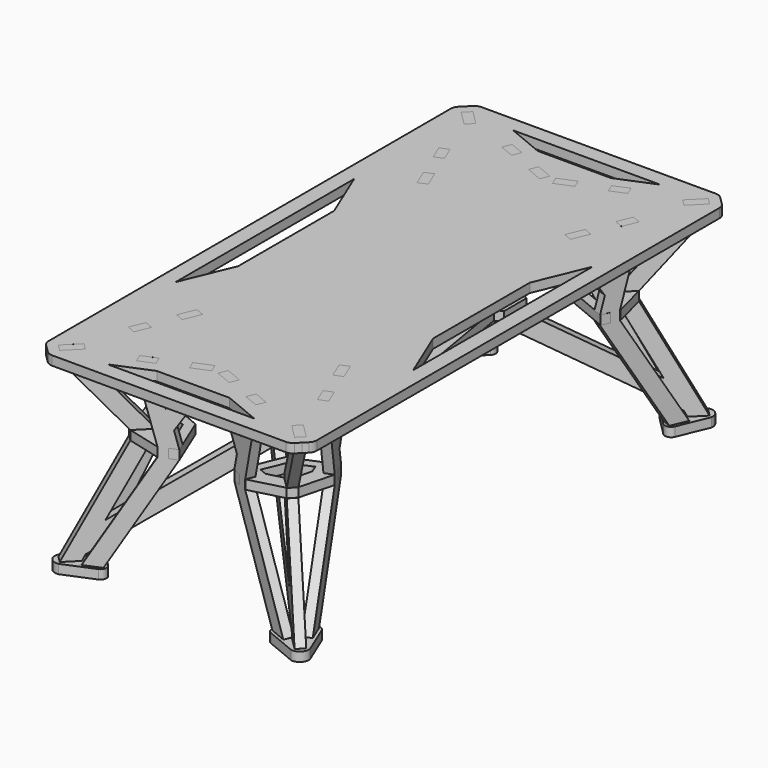
from build123d import *

# Parameters (mm, degrees)
F3_DEPTH  = 9.525
F6_DEPTH  = 9.525
F9_DEPTH  = 9.525
F12_DEPTH = 19.05
F15_DEPTH = 9.525
F18_DEPTH = 9.525
F21_DEPTH = 9.525
F24_DEPTH = 19.05
F25_DEPTH = 19.05
F26_DEPTH = 19.05
F27_DEPTH = 19.05
F28_DEPTH = 19.05
F31_DEPTH = 9.525
F34_DEPTH = 9.525
F37_DEPTH = 9.525
F40_DEPTH = 9.525
F43_DEPTH = 9.525
F46_DEPTH = 9.525
F49_DEPTH = 19.05
F52_DEPTH = 19.05
F55_DEPTH = 19.05
F58_DEPTH = 19.05


# Not quite as in the source:
# - a feature names something its author has since deleted; it is built from what else it names


with BuildPart() as f3:
    # F2 (on face) → F3 (new body, symmetric)
    with BuildSketch(Plane(origin=(0.1198709265, -0.1198709265, 0), x_dir=(0.7071067812, 0.7071067812, 0), z_dir=(0.7071067812, -0.7071067812, 0))):
        Polygon((72.1438338904, -0.0049185293), (72.1438338904, 19.0450814707), (76.4979425715, 19.0450814707), (82.66578851, 30.7838885104), (431.821256876, 234.9450814707), (431.821256876, 253.9950814707), (404.6548892498, 253.9950814707), (404.6548892498, 234.9450814707), (385.6048892498, 234.9450814707), (385.6048892498, 253.9950814707), (360.1152509125, 253.9950814707), (360.1152509125, 234.9450814707), (115.2544208988, 91.7679478036), (191.7653489945, 234.9450814707), (191.7653489945, 260.9125323174), (101.4276913023, 365.3266918993), (101.4276913023, 387.3450814707), (82.3776913023, 387.3450814707), (82.3776913023, 406.3950814707), (40.3938338904, 406.3950814707), (40.3938338904, 387.3450814707), (155.766372457, 253.9950814707), (173.7658607257, 253.9950814707), (173.7658607257, 234.9450814707), (155.766372457, 234.9450814707), (40.3938338904, 19.0450814707), (40.3938338904, -0.0049185293), align=None)
    extrude(amount=F3_DEPTH, both=True)


with BuildPart() as f6:
    # F5 (on line) → F6 (new body, symmetric)
    with BuildSketch(Plane(origin=(-6.0751025032, 14.6665948559, 0), x_dir=(-0.9238795325, -0.3826834324, 0), z_dir=(-0.3826834324, 0.9238795325, 0))):
        Polygon((-114.9103235555, 19.0475704348), (-109.7184195119, 19.0475704348), (-109.7184195119, -0.0024295652), (-77.970899542, -0.0024295652), (-77.970899542, 19.0475704348), (-206.3556462526, 234.9475704348), (-206.3556462526, 253.9975704348), (-170.8678305149, 387.3475704348), (-170.8678305149, 406.3975704348), (-203.7229094406, 406.3975704348), (-203.7229094406, 387.3475704348), (-210.0729094406, 387.3475704348), (-210.0729094406, 363.4866344375), (-220.3803230208, 324.7552114874), (-254.0578127939, 377.4178575907), (-254.0578127939, 387.3475704348), (-260.4078127939, 387.3475704348), (-260.4078127939, 406.3975704348), (-298.0948572889, 406.3975704348), (-298.0948572889, 387.3475704348), (-234.3391501722, 287.6505840032), (-243.2950702662, 253.9975704348), (-224.8253582594, 253.9975704348), (-224.8253582594, 234.9475704348), (-243.2950702662, 234.9475704348), align=None)
    extrude(amount=F6_DEPTH, both=True)


with BuildPart() as f9:
    # F8 (on line) → F9 (new body, symmetric)
    with BuildSketch(Plane(origin=(14.6666075026, -6.0751077416, 0), x_dir=(0.3826834324, 0.9238795325, 0), z_dir=(0.9238795325, -0.3826834324, 0))):
        Polygon((206.0561226085, 253.999334064), (206.0561226085, 234.949334064), (77.6713758978, 19.049334064), (77.6713758978, -0.000665936), (109.4188958678, -0.000665936), (109.4188958678, 19.049334064), (114.6107999114, 19.049334064), (242.995546622, 234.949334064), (224.5258346153, 234.949334064), (224.5258346153, 253.999334064), (242.995546622, 253.999334064), (234.039626528, 287.6523476325), (297.7953336448, 387.349334064), (297.7953336448, 406.399334064), (260.1082891497, 406.399334064), (260.1082891497, 387.349334064), (253.7582891497, 387.349334064), (253.7582891497, 377.41962122), (220.0807993766, 324.7569751166), (209.7733857965, 363.4883980668), (209.7733857965, 387.349334064), (203.4233857965, 387.349334064), (203.4233857965, 406.399334064), (170.5683068708, 406.399334064), (170.5683068708, 387.349334064), align=None)
    extrude(amount=F9_DEPTH, both=True)


with BuildPart() as f12:
    # F11 (on offset) → F12 (new body)
    with BuildSketch(Plane.XY.offset(234.9450814707)):
        Polygon((116.8785095215, 103.4081205726), (188.2171630859, 84.8387926817), (180.9265762568, 102.4385169148), (197.9916060299, 109.5076095697), (205.2830112566, 91.9059096972), (222.340834836, 98.9720172268), (186.3606104886, 185.829500883), (98.8556966186, 222.0692932606), (91.7885378003, 205.0048708916), (109.3906584881, 197.715026574), (102.3192360153, 180.6403091481), (84.721468389, 187.942802906), (103.4084260464, 116.8788522482), align=None)
        Polygon((142.3401087523, 128.8615316153), (129.6065747738, 116.1318197846), (116.1355222776, 129.6069170192), (128.8690562561, 142.3366288499), (120.4051498006, 174.5237104367), (126.7690426846, 189.8900208419), (171.7808899201, 171.2485534522), (190.1591339583, 126.8828481201), (174.639691322, 120.4540062485), align=None, mode=Mode.SUBTRACT)
    extrude(amount=F12_DEPTH)


with BuildPart() as f15:
    # F14 (on face) → F15 (new body, symmetric)
    with BuildSketch(Plane(origin=(279.3971066852, 279.3971066852, 0), x_dir=(-0.7071067812, 0.7071067812, 0), z_dir=(0.7071067812, 0.7071067812, 0))):
        Polygon((-323.8721739903, 0.0001450999), (-323.8721739903, 19.0501450999), (-319.5180653092, 19.0501450999), (-313.3502193707, 30.7889521396), (-9.531615302, 208.4403832929), (-9.531615302, 234.9501450999), (9.5219211653, 234.9501450999), (9.5219211653, 219.5815312562), (35.8052489953, 234.9501450999), (35.8052489953, 254.0001450999), (-35.9007569682, 254.0001450999), (-35.9007569682, 234.9501450999), (-280.7615869818, 91.7730114328), (-204.2506588862, 234.9501450999), (-204.2506588862, 260.9175959466), (-294.5883165784, 365.3317555285), (-294.5883165784, 387.3501450999), (-313.6383165784, 387.3501450999), (-313.6383165784, 406.4001450999), (-355.6221739903, 406.4001450999), (-355.6221739903, 387.3501450999), (-240.2496354237, 254.0001450999), (-222.2501471549, 254.0001450999), (-222.2501471549, 234.9501450999), (-240.2496354237, 234.9501450999), (-355.6221739903, 19.0501450999), (-355.6221739903, 0.0001450999), align=None)
    extrude(amount=F15_DEPTH, both=True)


with BuildPart() as f18:
    # F17 (on line) → F18 (new body, symmetric)
    with BuildSketch(Plane(origin=(462.3631726263, 191.5064043427, 0), x_dir=(-0.3826651956, 0.9238870862, 0), z_dir=(0.9238870862, 0.3826651956, 0))):
        Polygon((-7.6085330971, 254.0010976933), (-7.6085330971, 234.9510976933), (-135.9932798078, 19.0510976933), (-135.9932798078, 0.0010976933), (-104.2457598378, 0.0010976933), (-104.2457598378, 19.0510976933), (-99.0538557942, 19.0510976933), (29.3308909164, 234.9510976933), (10.8611789097, 234.9510976933), (10.8611789097, 254.0010976933), (29.3308909164, 254.0010976933), (20.3749708224, 287.6541112617), (84.1306779392, 387.3510976933), (84.1306779392, 406.4010976933), (46.4436334441, 406.4010976933), (46.4436334441, 387.3510976933), (40.0936334441, 387.3510976933), (40.0936334441, 377.4213848492), (6.416143671, 324.7587387459), (-3.8912699091, 363.490161696), (-3.8912699091, 387.3510976933), (-10.2412699091, 387.3510976933), (-10.2412699091, 406.4010976933), (-43.0963488348, 406.4010976933), (-43.0963488348, 387.3510976933), align=None)
    extrude(amount=F18_DEPTH, both=True)


with BuildPart() as f21:
    # F20 (on line) → F21 (new body, symmetric)
    with BuildSketch(Plane(origin=(87.9210659647, 212.1637274314, 0), x_dir=(0.9238179841, -0.3828319897, 0), z_dir=(-0.3828319897, -0.9238179841, 0))):
        Polygon((401.4962879207, 19.0500776933), (406.6881919643, 19.0500776933), (406.6881919643, 7.76933e-05), (438.4357119342, 7.76933e-05), (438.4357119342, 19.0500776933), (310.0509652236, 234.9500776933), (310.0509652236, 254.0000776933), (345.5387809613, 387.3500776933), (345.5387809613, 406.4000776933), (312.6837020356, 406.4000776933), (312.6837020356, 387.3500776933), (306.3337020356, 387.3500776933), (306.3337020356, 363.489141696), (296.0262884554, 324.7577187459), (262.3487986824, 377.4203648492), (262.3487986824, 387.3500776933), (255.9987986824, 387.3500776933), (255.9987986824, 406.4000776933), (218.3117541873, 406.4000776933), (218.3117541873, 387.3500776933), (282.067461304, 287.6530912617), (273.11154121, 254.0000776933), (291.5812532168, 254.0000776933), (291.5812532168, 234.9500776933), (273.11154121, 234.9500776933), align=None)
    extrude(amount=F21_DEPTH, both=True)


with BuildPart() as f24:
    # F23 (on offset) → F24 (new body)
    with BuildSketch(Plane.XY.offset(234.9501450999)):
        Polygon((455.509489859, 116.7611451179), (474.0788177498, 188.0997986823), (456.4790935167, 180.8092118531), (449.4100008618, 197.8742416263), (467.0117007343, 205.165646853), (459.9455932048, 222.2234704324), (373.0881095486, 186.243246085), (336.8483171709, 98.7383322149), (353.9127395399, 91.6711733967), (361.2025838575, 109.2732940845), (378.2773012834, 102.2018716117), (370.9748075255, 84.6041039854), (442.0387581833, 103.2910616427), align=None)
        Polygon((430.0560788163, 142.2227443486), (442.7857906469, 129.4892103702), (429.3106934123, 116.018157874), (416.5809815817, 128.7516918524), (384.3938999948, 120.2877853969), (369.0275895896, 126.651678281), (387.6690569793, 171.6635255165), (432.0347623114, 190.0417695547), (438.4636041831, 174.5223269184), align=None, mode=Mode.SUBTRACT)
    extrude(amount=F24_DEPTH)


with BuildPart() as f25:
    # F0 (on Top) → F25 (new body)
    with BuildSketch(Plane.XY):
        with BuildLine():
            Line((103.8517784432, 62.0606233049), (62.0501863777, 103.7966362254))
            ThreePointArc((62.0501863777, 103.7966362254), (50.6222299212, 107.3273041247), (41.3345954203, 99.790484506))
            Line((41.3345954203, 99.790484506), (15.7147154747, 37.7569687534))
            ThreePointArc((15.7147154747, 37.7569687534), (20.9923055548, 20.8615847055), (37.8937751532, 15.6035161825))
            Line((37.8937751532, 15.6035161825), (99.8533848211, 41.3606347628))
            ThreePointArc((99.8533848211, 41.3606347628), (107.3873805868, 50.6415315899), (103.8517784432, 62.0606233049))
        make_face()
        Polygon((35.3410425095, 21.7441998811), (21.8706744367, 35.2145539371), (44.3213147394, 57.6651942398), (57.7916758038, 44.1948331754), align=None, mode=Mode.SUBTRACT)
        Polygon((35.5910924595, 69.3310921079), (47.741291437, 98.6642672651), (65.3411965314, 91.3741478786), (53.1909975538, 62.0409727213), align=None, mode=Mode.SUBTRACT)
        Polygon((91.6462977705, 65.4539098912), (98.936417157, 47.8540047968), (69.5988084838, 35.7019693968), (62.3086890973, 53.3018744911), align=None, mode=Mode.SUBTRACT)
    extrude(amount=F25_DEPTH)


with BuildPart() as f26:
    # F0 (on Top) → F26 (new body)
    with BuildSketch(Plane.XY):
        with BuildLine():
            Line((496.8432117084, 103.7402135395), (455.0267768688, 61.9770459526))
            ThreePointArc((455.0267768688, 61.9770459526), (451.5142547987, 50.5275807617), (459.0848956853, 41.2478468746))
            ThreePointArc((459.0848956853, 41.2478468746), (459.115702577, 41.2350329946), (459.1465430272, 41.2223000948))
            Line((459.1465430272, 41.2223000948), (521.8248655775, 15.2482799444))
            ThreePointArc((521.8248655775, 15.2482799444), (538.191689524, 20.6006442335), (543.556206165, 36.9634890592))
            Line((543.556206165, 36.9634890592), (517.7368995388, 99.3002895837))
            Line((517.7368995388, 99.3002895837), (517.4423179946, 100.011512051))
            ThreePointArc((517.4423179946, 100.011512051), (508.1237343014, 107.2952008746), (496.8432117084, 103.7402135395))
        make_face()
        Polygon((489.404191899, 35.5571192782), (460.0729709053, 47.7120349513), (467.3098559279, 65.1754776945), (496.6410769216, 53.0205620214), align=None, mode=Mode.SUBTRACT)
        Polygon((537.7076836736, 34.541086975), (524.2381294154, 21.0717654255), (501.7874891128, 43.5224057281), (515.2578732944, 56.9927899097), align=None, mode=Mode.SUBTRACT)
        Polygon((493.4490156942, 91.5631395448), (511.0490646865, 98.8529115212), (523.1992132676, 69.5182202606), (505.5991642753, 62.2284482841), align=None, mode=Mode.SUBTRACT)
    extrude(amount=F26_DEPTH)


with BuildPart() as f27:
    # F0 (on Top) → F27 (new body)
    with BuildSketch(Plane.XY):
        with BuildLine():
            Line((99.729697681, 1076.290326866), (37.2638967919, 1102.1180850915))
            ThreePointArc((37.2638967919, 1102.1180850915), (20.8268547426, 1096.7789895039), (15.4792253934, 1080.3447218485))
            Line((15.4792253934, 1080.3447218485), (41.3295247664, 1017.861248421))
            ThreePointArc((41.3295247664, 1017.861248421), (50.6004156209, 1010.2487394776), (62.0794812799, 1013.7316637153))
            Line((62.0794812799, 1013.7316637153), (103.866883956, 1055.5379496472))
            Line((103.866883956, 1055.5379496472), (103.9049132936, 1055.5759961698))
            ThreePointArc((103.9049132936, 1055.5759961698), (107.3599726929, 1067.0229131057), (99.7794096849, 1076.269772425))
            Line((99.7794096849, 1076.269772425), (99.729697681, 1076.290326866))
        make_face()
        Polygon((65.4208716795, 1026.0711758783), (47.8178602661, 1018.7885603331), (35.6801676907, 1048.1269126887), (53.2831791041, 1055.409528234), align=None, mode=Mode.SUBTRACT)
        Polygon((43.825407668, 1060.3338990517), (21.3734913956, 1082.7832633121), (34.8359362826, 1096.2459340352), (57.2861657843, 1073.7961873681), align=None, mode=Mode.SUBTRACT)
        Polygon((70.7823829162, 1081.3877981223), (100.1232616549, 1069.256213937), (92.8443111437, 1051.6516866938), (63.5034324051, 1063.7832708791), align=None, mode=Mode.SUBTRACT)
    extrude(amount=F27_DEPTH)


with BuildPart() as f28:
    # F0 (on Top) → F28 (new body)
    with BuildSketch(Plane.XY):
        with BuildLine():
            Line((517.5915767567, 1017.7489309873), (543.5403541426, 1080.3696806001))
            ThreePointArc((543.5403541426, 1080.3696806001), (538.1610200159, 1096.7468930862), (521.7742455342, 1102.0970282758))
            Line((521.7742455342, 1102.0970282758), (459.1805971498, 1076.1780060223))
            Line((459.1805971498, 1076.1780060223), (459.0026242216, 1076.1043102975))
            ThreePointArc((459.0026242216, 1076.1043102975), (451.5153222415, 1066.912204013), (454.9120530441, 1055.5536509035))
            Line((454.9120530441, 1055.5536509035), (455.0482408698, 1055.4174220551))
            Line((455.0482408698, 1055.4174220551), (496.8306038614, 1013.6224733009))
            Line((496.8306038614, 1013.6224733009), (496.8633947836, 1013.5896725014))
            ThreePointArc((496.8633947836, 1013.5896725014), (508.3163354223, 1010.1250092731), (517.5738216828, 1017.7060836492))
            Line((517.5738216828, 1017.7060836492), (517.5915767567, 1017.7489309873))
        make_face()
        Polygon((467.3629129365, 1052.0746695321), (460.0747414799, 1069.6753813592), (489.4092611916, 1081.8223337869), (496.6974326482, 1064.2216219599), align=None, mode=Mode.SUBTRACT)
        Polygon((523.2513883009, 1047.9951071094), (511.0970260539, 1018.663656781), (493.4981558568, 1025.9562741293), (505.6525181039, 1055.2877244577), align=None, mode=Mode.SUBTRACT)
        Polygon((501.7279177318, 1073.8354100465), (524.1818351597, 1096.2827727456), (537.6502567338, 1082.8104183331), (515.1963353513, 1060.3630595898), align=None, mode=Mode.SUBTRACT)
    extrude(amount=F28_DEPTH)


with BuildPart() as f31:
    # F30 (on face) → F31 (new body, symmetric)
    with BuildSketch(Plane(origin=(558.7970964269, 558.8606196936, 0), x_dir=(-0.7071469692, 0.7070665909, 0), z_dir=(0.7070665909, 0.7071469692, 0))):
        Polygon((385.3406808672, 234.9501287292), (404.3942173345, 234.9501287292), (404.3942173345, 208.4403669221), (708.2128214032, 30.7889357689), (714.3806673417, 19.0501287292), (718.7347760228, 19.0501287292), (718.7347760228, 0.0001287292), (750.4847760228, 0.0001287292), (750.4847760228, 19.0501287292), (635.1122374562, 234.9501287292), (617.1127491875, 234.9501287292), (617.1127491875, 254.0001287292), (635.1122374562, 254.0001287292), (750.4847760228, 387.3501287292), (750.4847760228, 406.4001287292), (708.5009186109, 406.4001287292), (708.5009186109, 387.3501287292), (689.425110817, 387.3501287292), (689.425110817, 365.3019099682), (599.1132609187, 260.9175795759), (599.1132609187, 234.9501287292), (675.6241890144, 91.7729950621), (430.7633590007, 234.9501287292), (430.7633590007, 254.0001287292), (359.0573530372, 254.0001287292), (359.0573530372, 234.9501287292), (385.3406808672, 219.5815148854), align=None)
    extrude(amount=F31_DEPTH, both=True)


with BuildPart() as f34:
    # F33 (on line) → F34 (new body, symmetric)
    with BuildSketch(Plane(origin=(409.5199129468, 169.4241976029, 0), x_dir=(-0.3822895299, 0.9240425939, 0), z_dir=(0.9240425939, 0.3822895299, 0))):
        Polygon((917.9344551891, 19.0510976933), (923.1263592327, 19.0510976933), (923.1263592327, 0.0010976933), (954.8738792027, 0.0010976933), (954.8738792027, 19.0510976933), (826.489132492, 234.9510976933), (826.489132492, 254.0010976933), (861.9769482298, 387.3510976933), (861.9769482298, 406.4010976933), (829.121869304, 406.4010976933), (829.121869304, 387.3510976933), (822.773873806, 387.3510976933), (822.773873806, 363.4976938682), (812.4644557239, 324.7587387459), (778.7790298462, 377.4337948082), (778.7790298462, 387.3510976933), (772.4369659508, 387.3510976933), (772.4369659508, 406.4010976933), (734.7499214558, 406.4010976933), (734.7499214558, 387.3510976933), (798.5056285725, 287.6541112617), (789.5497084785, 254.0010976933), (808.0194204853, 254.0010976933), (808.0194204853, 234.9510976933), (789.5497084785, 234.9510976933), align=None)
    extrude(amount=F34_DEPTH, both=True)


with BuildPart() as f37:
    # F36 (on line) → F37 (new body, symmetric)
    with BuildSketch(Plane(origin=(388.5374554756, 939.698409741, 0), x_dir=(-0.924122165, 0.3820971397, 0), z_dir=(0.3820971397, 0.924122165, 0))):
        Polygon((310.8441225105, 19.0495613225), (316.0360265541, 19.0495613225), (316.0360265541, -0.0004386775), (347.7835465241, -0.0004386775), (347.7835465241, 19.0495613225), (219.3987998134, 234.9495613225), (219.3987998134, 253.9995613225), (254.8866155511, 387.3495613225), (254.8866155511, 406.3995613225), (222.0315366254, 406.3995613225), (222.0315366254, 387.3495613225), (215.6789898872, 387.3495613225), (215.6789898872, 363.4790556313), (205.3741230453, 324.7572023751), (171.7055737972, 377.4058678727), (171.7055737972, 387.3495613225), (165.3466332722, 387.3495613225), (165.3466332722, 406.3995613225), (127.6595887772, 406.3995613225), (127.6595887772, 387.3495613225), (191.4152958939, 287.652574891), (182.4593757999, 253.9995613225), (200.9290878066, 253.9995613225), (200.9290878066, 234.9495613225), (182.4593757999, 234.9495613225), align=None)
    extrude(amount=F37_DEPTH, both=True)


with BuildPart() as f40:
    # F39 (on face) → F40 (new body, symmetric)
    with BuildSketch(Plane(origin=(-279.3619916801, 279.4438619945, 0), x_dir=(0.7072103714, 0.7070031758, 0), z_dir=(0.7070031758, -0.7072103714, 0))):
        Polygon((1109.6777865613, 19.0498950999), (1114.0318952424, 19.0498950999), (1114.0318952424, -0.0001049001), (1145.7818952424, -0.0001049001), (1145.7818952424, 19.0498950999), (1030.4093566758, 234.9498950999), (1012.4098684071, 234.9498950999), (1012.4098684071, 253.9998950999), (1030.4093566758, 253.9998950999), (1145.7818952424, 387.3498950999), (1145.7818952424, 406.3998950999), (1103.7980378305, 406.3998950999), (1103.7980378305, 387.3498950999), (1084.7434997559, 387.3498950999), (1084.7434997559, 365.3262603266), (994.4103801383, 260.9173459466), (994.4103801383, 234.9498950999), (1070.921308234, 91.7727614328), (826.0604782204, 234.9498950999), (826.0604782204, 253.9998950999), (800.570839883, 253.9998950999), (800.570839883, 234.9498950999), (781.520839883, 234.9498950999), (781.520839883, 253.9998950999), (754.3544722568, 253.9998950999), (754.3544722568, 234.9498950999), (1103.5099406228, 30.7887021396), align=None)
    extrude(amount=F40_DEPTH, both=True)


with BuildPart() as f43:
    # F42 (on line) → F43 (new body, symmetric)
    with BuildSketch(Plane(origin=(-307.1191658231, 741.6834203732, 0), x_dir=(0.9239218807, 0.3825811788, 0), z_dir=(0.3825811788, -0.9239218807, 0))):
        Polygon((829.1215476453, 19.0500713225), (834.3134516889, 19.0500713225), (834.3134516889, 7.13225e-05), (866.0609716588, 7.13225e-05), (866.0609716588, 19.0500713225), (737.6762249482, 234.9500713225), (737.6762249482, 254.0000713225), (773.1640406859, 387.3500713225), (773.1640406859, 406.4000713225), (740.3089617602, 406.4000713225), (740.3089617602, 387.3500713225), (733.9589595795, 387.3500713225), (733.9589595795, 363.489127131), (723.65154818, 324.7577123751), (689.981341362, 377.4089698718), (689.981341362, 387.3500713225), (683.6240584069, 387.3500713225), (683.6240584069, 406.4000713225), (645.9370139119, 406.4000713225), (645.9370139119, 387.3500713225), (709.6927210286, 287.653084891), (700.7368009346, 254.0000713225), (719.2065129414, 254.0000713225), (719.2065129414, 234.9500713225), (700.7368009346, 234.9500713225), align=None)
    extrude(amount=F43_DEPTH, both=True)


with BuildPart() as f46:
    # F45 (on line) → F46 (new body, symmetric)
    with BuildSketch(Plane(origin=(67.1436506911, -27.8229764964, 0), x_dir=(0.382814559, 0.9238252072, 0), z_dir=(0.9238252072, -0.382814559, 0))):
        Polygon((1131.5330661809, 19.0503213225), (1136.7249702245, 19.0503213225), (1136.7249702245, 0.0003213225), (1168.4724901944, 0.0003213225), (1168.4724901944, 19.0503213225), (1040.0877434837, 234.9503213225), (1040.0877434837, 254.0003213225), (1075.5755592215, 387.3503213225), (1075.5755592215, 406.4003213225), (1042.7204802958, 406.4003213225), (1042.7204802958, 387.3503213225), (1036.3608598709, 387.3503213225), (1036.3608598709, 363.4532353503), (1026.0630667156, 324.7579623751), (992.3783540726, 377.431903128), (992.3783540726, 387.3503213225), (986.0355769425, 387.3503213225), (986.0355769425, 406.4003213225), (948.3485324475, 406.4003213225), (948.3485324475, 387.3503213225), (1012.1042395642, 287.653334891), (1003.1483194702, 254.0003213225), (1021.618031477, 254.0003213225), (1021.618031477, 234.9503213225), (1003.1483194702, 234.9503213225), align=None)
    extrude(amount=F46_DEPTH, both=True)


with BuildPart() as f49:
    # F48 (on offset) → F49 (new body)
    with BuildSketch(Plane.XY.offset(234.9501287292)):
        Polygon((104.2109857346, 999.9368687937), (85.6416578438, 928.5982152292), (103.2413820769, 935.8888020584), (110.3104747318, 918.8237722853), (92.7087748593, 911.5323670586), (99.7748823888, 894.4745434792), (186.632366045, 930.4547678265), (222.8721584227, 1017.9596816966), (205.8077360536, 1025.0268405149), (198.5178917361, 1007.424719827), (181.4431743102, 1014.4961422998), (188.7456680681, 1032.0939099261), (117.6817174103, 1013.4069522688), align=None)
        Polygon((129.6643967773, 974.4752695629), (116.9346849467, 987.2088035414), (130.4097821813, 1000.6798560376), (143.1394940119, 987.9463220591), (175.3265755987, 996.4102285146), (190.692886004, 990.0463356306), (172.0514186143, 945.0344883951), (127.6857132822, 926.6562443569), (121.2568714105, 942.1756869931), align=None, mode=Mode.SUBTRACT)
    extrude(amount=F49_DEPTH)


with BuildPart() as f52:
    # F51 (on offset) → F52 (new body)
    with BuildSketch(Plane.XY.offset(234.9498950999)):
        Polygon((442.4701955485, 1014.9229667504), (371.131541984, 1033.4922946413), (378.4221288132, 1015.8925704081), (361.35709904, 1008.8234777533), (354.0656938134, 1026.4251776258), (337.007870234, 1019.3590700962), (372.9880945813, 932.50158644), (460.4930084514, 896.2617940624), (467.5601672696, 913.3262164314), (449.9580465818, 920.616060749), (457.0294690546, 937.6907781749), (474.6272366809, 930.388284417), (455.9402790236, 1001.4522350748), align=None)
        Polygon((417.0085963177, 989.4695557077), (429.7421302962, 1002.1992675384), (443.2131827924, 988.7241703038), (430.4796488139, 975.9944584731), (438.9435552694, 943.8073768863), (432.5796623853, 928.4410664811), (387.5678151499, 947.0825338708), (369.1895711117, 991.4482392029), (384.7090137479, 997.8770810745), align=None, mode=Mode.SUBTRACT)
    extrude(amount=F52_DEPTH)


with BuildPart() as f55:
    # F54 (on offset) → F55 (new body)
    with BuildSketch(Plane.XY.offset(254.0001450999)):
        Polygon((229.4062823057, 867.0365809124), (229.4062823057, 809.1738861036), (244.6239178905, 800.3879801023), (203.3169243548, 558.9507038395), (244.1765100053, 316.7285120233), (229.4286527446, 308.2138326639), (229.4286527446, 250.3511378551), (279.5392163804, 221.4197904507), (329.6497800163, 250.3511378551), (329.6497800163, 308.2138326639), (315.2171087009, 316.546539333), (355.7167675282, 559.1693375004), (314.7207803598, 800.5675397122), (329.6274095774, 809.1738861036), (329.6274095774, 867.0365809124), (304.9168459415, 881.3032314794), (279.5168459415, 895.9679283168), (254.1168459415, 881.3032314794), align=None)
        Polygon((298.0475306041, 247.2727716594), (279.5168459415, 265.8051252365), (261.4959180355, 247.7835118771), (248.0230078666, 261.2559096028), (266.0434320351, 279.2770192055), (247.3390046986, 297.9807351177), (260.8133450947, 311.4555880307), (279.5168459415, 292.7527985729), (298.7271042289, 311.9637875516), (312.2027993105, 298.488605019), (292.9919442111, 279.2770192055), (311.5219573157, 260.7477108913), align=None, mode=Mode.SUBTRACT)
        Polygon((272.2180339866, 341.3720666942), (235.5218205917, 558.913118527), (272.7169232031, 776.3166014757), (279.5168459415, 780.2425386992), (286.6692053774, 776.1131220536), (323.5198840888, 559.1238944336), (287.2050077294, 341.5710267672), (279.5392163804, 337.1451800683), align=None, mode=Mode.SUBTRACT)
        Polygon((298.0182122612, 806.1009859618), (279.4875275987, 824.633339539), (261.4665996926, 806.6117261795), (247.9936895237, 820.0841239053), (266.0141136922, 838.105233508), (247.3096863558, 856.8089494201), (260.7840267518, 870.2838023332), (279.4875275987, 851.5810128754), (298.6977858859, 870.7920018541), (312.1734809676, 857.3168193215), (292.9626258682, 838.105233508), (311.4926389728, 819.5759251938), align=None, mode=Mode.SUBTRACT)
    extrude(amount=-F55_DEPTH)


with BuildPart() as f58:
    # F57 (on offset) → F58 (new body)
    with BuildSketch(Plane.XY.offset(387.35)):
        with BuildLine():
            Line((536.4708682518, 5.608798301), (544.8278111014, 13.96560249))
            Line((544.8278111014, 13.96560249), (553.2187870188, 22.3564391822))
            ThreePointArc((553.2187870188, 22.3564391822), (557.3480914419, 28.5360233313), (558.798514527, 35.825377771))
            Line((558.798514527, 35.825377771), (558.8159444372, 249.0342241186))
            Line((558.8159444372, 249.0342241186), (558.8412616174, 558.7229554382))
            Line((558.8412616174, 558.7229554382), (558.8665891192, 868.5379441028))
            Line((558.8665891192, 868.5379441028), (558.8840086917, 1081.6203358468))
            ThreePointArc((558.8840086917, 1081.6203358468), (557.4347130247, 1088.9100829003), (553.3062453568, 1095.0904246991))
            Line((553.3062453568, 1095.0904246991), (544.9171263965, 1103.4818514446))
            Line((544.9171263965, 1103.4818514446), (536.535572746, 1111.8657107992))
            ThreePointArc((536.535572746, 1111.8657107992), (530.3545081901, 1115.996648324), (523.0629950551, 1117.4471792891))
            Line((523.0629950551, 1117.4471792891), (442.6557703542, 1117.4457396011))
            Line((442.6557703542, 1117.4457396011), (116.5401726367, 1117.439900515))
            Line((116.5401726367, 1117.439900515), (35.9818336035, 1117.4384581213))
            ThreePointArc((35.9818336035, 1117.4384581213), (28.691405812, 1115.9880941753), (22.5110375085, 1111.858089261))
            Line((22.5110375085, 1111.858089261), (14.1245930875, 1103.4707071465))
            Line((14.1245930875, 1103.4707071465), (5.7539980097, 1095.0991761474))
            ThreePointArc((5.7539980097, 1095.0991761474), (1.6230715906, 1088.9144511114), (0.1751379356, 1081.619325))
            Line((0.1751379356, 1081.619325), (0.2897951617, 867.8994070639))
            Line((0.2897951617, 867.8994070639), (0.4556632505, 558.7229554382))
            Line((0.4556632505, 558.7229554382), (0.6210733684, 250.4001569316))
            Line((0.6210733684, 250.4001569316), (0.7359240206, 36.3196948664))
            ThreePointArc((0.7359240206, 36.3196948664), (2.1896029963, 29.0311421797), (6.321559068, 22.8535114159))
            Line((6.321559068, 22.8535114159), (14.7167911679, 14.4657805079))
            Line((14.7167911679, 14.4657805079), (23.1566134063, 6.0334993029))
            ThreePointArc((23.1566134063, 6.0334993029), (29.3269986718, 1.9115960183), (36.6041100069, 0.4599102298))
            Line((36.6041100069, 0.4599102298), (117.0948497032, 0.3886490224))
            Line((117.0948497032, 0.3886490224), (279.8062461273, 0.2445950528))
            Line((279.8062461273, 0.2445950528), (442.0765385642, 0.1009316076))
            Line((442.0765385642, 0.1009316076), (522.9837302131, 0.029301701))
            ThreePointArc((522.9837302131, 0.029301701), (530.2828505794, 1.4761335623), (536.4708682518, 5.608798301))
        make_face()
        Polygon((35.4171507061, 21.7072200031), (28.6784371567, 28.4399124701), (21.9397236074, 35.1726049372), (51.6342891533, 64.8664979284), (65.1055425406, 51.3949394227), align=None, mode=Mode.SUBTRACT)
        Polygon((71.1389556527, 155.153170228), (83.7128162384, 185.5104416609), (101.3146438778, 178.2198349514), (88.7407832921, 147.8625635185), align=None, mode=Mode.SUBTRACT)
        Polygon((123.0062693357, 230.5872142315), (105.4048389196, 237.877741456), (119.8273196894, 272.6977598), (137.4287501055, 265.4072325755), align=None, mode=Mode.SUBTRACT)
        Polygon((178.4952230677, 101.4295413492), (185.7863515615, 83.8272720575), (155.4313004017, 71.253746748), (148.1401719078, 88.8560160396), align=None, mode=Mode.SUBTRACT)
        Polygon((238.1548136473, 105.517603457), (230.8638393879, 123.1202483177), (265.6831938015, 137.5423433362), (272.9741680609, 119.9396984754), align=None, mode=Mode.SUBTRACT)
        Polygon((431.7855853832, 31.8600557655), (279.8062461273, 31.9946082775), (127.3507526973, 32.1295823451), (203.6897280957, 63.7503506391), (279.8062461273, 63.7503506391), (354.8300109414, 63.7503506391), align=None, mode=Mode.SUBTRACT)
        Polygon((328.0688524246, 122.9611486197), (320.7723498344, 105.3577661514), (285.950429751, 119.7912553142), (293.2469323412, 137.3946377825), align=None, mode=Mode.SUBTRACT)
        Polygon((410.7838869095, 88.6807963252), (403.4902155399, 71.080185473), (373.1353270356, 83.6592137277), (380.4289984051, 101.2598245799), align=None, mode=Mode.SUBTRACT)
        Polygon((507.9074338642, 64.3577784927), (537.595629692, 34.6690900625), (530.8600366115, 27.9336087407), (524.124443531, 21.1981274188), (494.4362477032, 50.8868158491), align=None, mode=Mode.SUBTRACT)
        Polygon((487.6554608345, 155.3352326155), (470.0540304184, 148.0446010828), (457.4803051266, 178.4007574464), (475.0817355427, 185.691388979), align=None, mode=Mode.SUBTRACT)
        Polygon((453.3914923668, 238.0599677563), (435.7899129391, 230.7697236538), (421.3679065423, 265.5902437258), (438.96948597, 272.8804878283), align=None, mode=Mode.SUBTRACT)
        Polygon((32.3300069293, 326.9546461271), (32.2056670376, 558.7229554382), (32.0810221122, 791.0598445022), (76.6922682524, 683.2342282061), (76.6922682524, 558.7229554382), (76.6922682524, 434.0579092698), align=None, mode=Mode.SUBTRACT)
        Polygon((105.4228395224, 879.5479536057), (123.0274066329, 886.8315815926), (137.4360616352, 852.0057867529), (119.8314945247, 844.722158766), align=None, mode=Mode.SUBTRACT)
        Polygon((71.1927935481, 962.2863531113), (88.797301054, 969.5698618889), (101.3586799895, 939.2085488864), (83.7541724836, 931.9250401088), align=None, mode=Mode.SUBTRACT)
        Polygon((21.3576905829, 1082.7672708355), (28.0932642719, 1089.5035976332), (34.828837961, 1096.2399244308), (64.5183697343, 1066.5537118912), (51.0482574281, 1053.0800233397), align=None, mode=Mode.SUBTRACT)
        Polygon((156.6300839186, 1045.8927154541), (186.9934499264, 1033.3383083344), (179.7140230981, 1015.732705855), (149.3506570903, 1028.2871129748), align=None, mode=Mode.SUBTRACT)
        Polygon((232.0956284897, 994.0736069456), (239.3758296967, 1011.6800069809), (274.2054686171, 997.2780407187), (266.9252674102, 979.6716406834), align=None, mode=Mode.SUBTRACT)
        Polygon((527.1103282608, 791.9035339722), (527.0912656534, 558.7229554382), (527.0722139981, 325.6763481411), (482.5911819935, 433.0714376402), (482.5911819935, 558.7229554382), (482.5911819935, 684.4696478189), align=None, mode=Mode.SUBTRACT)
        Polygon((320.8523145956, 1012.0268094132), (328.1411622981, 994.4243449195), (293.3191323493, 980.0052007664), (286.0302846469, 997.60766526), align=None, mode=Mode.SUBTRACT)
        Polygon((279.8064692498, 1053.9086340066), (203.7182529082, 1053.9086340066), (126.8536027401, 1085.6900284369), (432.3702368457, 1085.6954986995), (355.606153285, 1053.9099911967), align=None, mode=Mode.SUBTRACT)
        Polygon((380.5114260915, 1016.1093815505), (373.2223642994, 1033.7129434392), (403.5800827671, 1046.2830861852), (410.8691445592, 1028.6795242965), align=None, mode=Mode.SUBTRACT)
        Polygon((435.8119317879, 886.7493213649), (453.4129798412, 879.4556856155), (438.9847517013, 844.6373939514), (421.383703648, 851.9310297008), align=None, mode=Mode.SUBTRACT)
        Polygon((470.0897336006, 969.4703221321), (487.6898229122, 962.174475193), (475.1047803444, 931.8150289172), (457.5046910328, 939.1108758563), align=None, mode=Mode.SUBTRACT)
        Polygon((524.2126931626, 1096.2523568463), (530.9473151898, 1089.5158821739), (537.681937217, 1082.7794075014), (507.9898238176, 1053.0954599387), (494.516044191, 1066.5638749589), align=None, mode=Mode.SUBTRACT)
    extrude(amount=F58_DEPTH)


solid = Compound([f3.part, f6.part, f9.part, f12.part, f15.part, f18.part, f21.part, f24.part, f25.part, f26.part, f27.part, f28.part, f31.part, f34.part, f37.part, f40.part, f43.part, f46.part, f49.part, f52.part, f55.part, f58.part])
